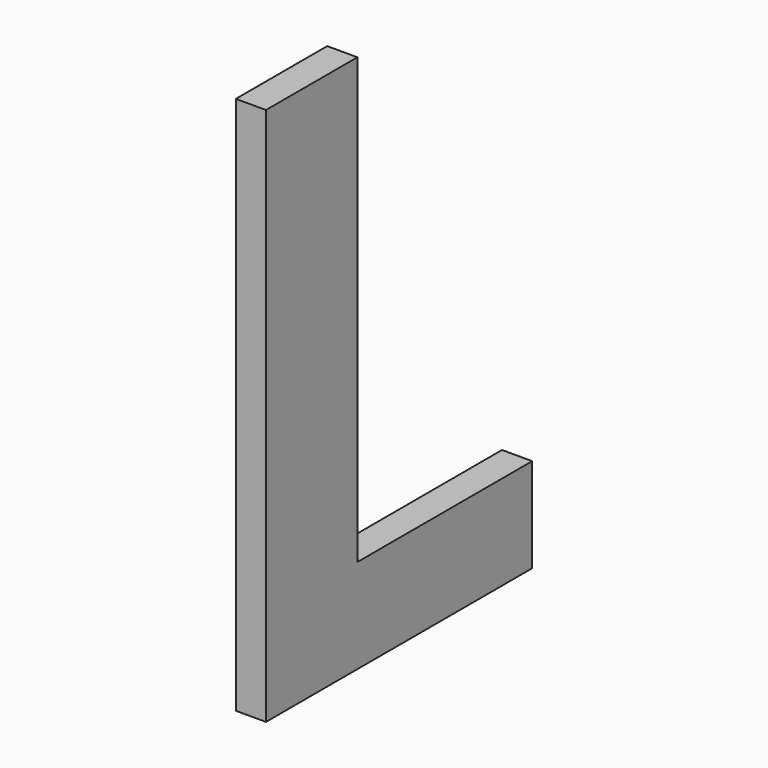
from build123d import *

# Parameters (mm, degrees)
F0_TEXT_SIZE = 635
F1_DEPTH     = 12.7


# Not quite as in the source:
# - Text() gives the source's letters only with a copy of the font that has no kerning and outlines rounded to 1/6400 em; it was checked with that copy


with BuildPart() as f1:
    # F0 (on Right) → F1 (new body, symmetric)
    with BuildSketch(Plane.YZ):
        with Locations((-229.4529980121, -226.0410247056)):
            Text('L', F0_TEXT_SIZE, font='Open Sans', font_style=FontStyle.BOLD, text_align=(TextAlign.LEFT, TextAlign.BOTTOM))
    extrude(amount=F1_DEPTH, both=True)


solid = f1.part
